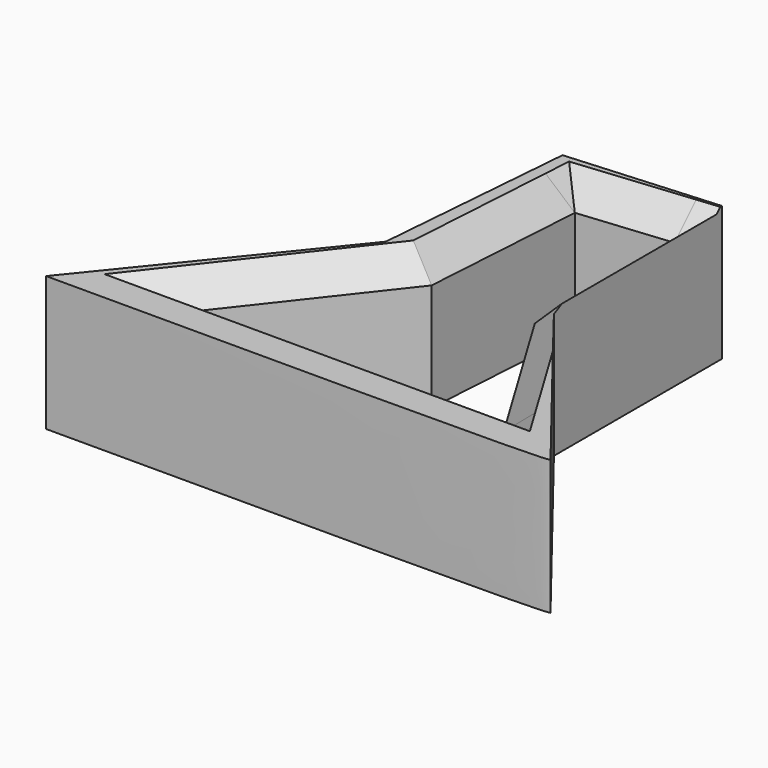
from build123d import *

# Parameters (mm, degrees)
F1_DEPTH     = 25.4
F3_DEPTH     = 50.8
F5_T4_DEPTH  = 64.0057067986
F5_T9_DEPTH  = 86.9283653755
F5_T15_DEPTH = 60.9737188004
F5_T20_DEPTH = 59.1061688919
F5_T25_DEPTH = 43.6640606018
F5_T31_DEPTH = 57.4502846001


# Not quite as in the source:
# - a fillet or chamfer that OpenCascade refuses, or shapes differently, is made with other operations: its cross-section is extruded or revolved along the edge and cut away or added
# - a feature of the source that left no trace in its solid (it failed there, or was rolled back) is left out


with BuildPart() as f1:
    # F0 (on Top) → F1 (new body)
    with BuildSketch(Plane.XY):
        with BuildLine():
            add(Edge.make_bspline(
                [(-48.315115273, -59.7526505589), (-37.5784229901, -46.4742837681), (-26.8417307072, -33.1959169772), (-16.1050384243, -19.9175501863)],
                knots=[0, 0, 0, 0, 51.2281589782, 51.2281589782, 51.2281589782, 51.2281589782], degree=3))
            add(Edge.make_bspline(
                [(-48.315115273, -59.7526505589), (-1.0274761031, -59.7958142001), (46.2601630669, -59.8389778412), (46.3316738605, -59.1182820499)],
                knots=[0, 0, 0, 0, 0.8911107377, 0.8911107377, 0.8911107377, 0.8911107377], degree=3))
            add(Edge.make_bspline(
                [(46.3316738605, -59.1182820499), (46.3235373894, -59.1079000767), (46.3154009182, -59.0975181035), (46.3072644471, -59.0871361303)],
                knots=[0, 0, 0, 0, 0.0395712999, 0.0395712999, 0.0395712999, 0.0395712999], degree=3))
            add(Edge.make_bspline(
                [(46.3072644471, -59.0871361303), (36.0194733937, -45.9601220924), (25.7316823403, -32.8331080545), (15.4438912868, -19.7060940166)],
                knots=[0.0395712999, 0.0395712999, 0.0395712999, 0.0395712999, 50.0737024584, 50.0737024584, 50.0737024584, 50.0737024584], degree=3))
            add(Edge.make_bspline(
                [(15.4438912868, -19.7060940166), (10.2959275246, -13.1373960111), (5.1479637623, -6.5686980055), (0, 0)],
                knots=[50.0737024584, 50.0737024584, 50.0737024584, 50.0737024584, 75.1105536876, 75.1105536876, 75.1105536876, 75.1105536876], degree=3))
            add(Edge.make_bspline(
                [(-16.1050384243, -19.9175501863), (-10.7366922829, -13.2783667909), (-5.3683461414, -6.6391833954), (0, 0)],
                knots=[51.2281589782, 51.2281589782, 51.2281589782, 51.2281589782, 76.8422384673, 76.8422384673, 76.8422384673, 76.8422384673], degree=3))
        make_face()
        with BuildLine():
            add(Edge.make_bspline(
                [(-16.1050384243, -19.9175501863), (-15.0708617229, -7.3149574714), (-14.0366850214, 5.2876352436), (-13.0025083199, 17.8902279586)],
                knots=[0, 0, 0, 0, 37.9348623472, 37.9348623472, 37.9348623472, 37.9348623472], degree=3))
            add(Edge.make_bspline(
                [(-16.1050384243, -19.9175501863), (-10.7366922829, -13.2783667909), (-5.3683461414, -6.6391833954), (0, 0)],
                knots=[51.2281589782, 51.2281589782, 51.2281589782, 51.2281589782, 76.8422384673, 76.8422384673, 76.8422384673, 76.8422384673], degree=3))
            add(Edge.make_bspline(
                [(15.4438912868, -19.7060940166), (10.2959275246, -13.1373960111), (5.1479637623, -6.5686980055), (0, 0)],
                knots=[50.0737024584, 50.0737024584, 50.0737024584, 50.0737024584, 75.1105536876, 75.1105536876, 75.1105536876, 75.1105536876], degree=3))
            add(Edge.make_bspline(
                [(15.4438912868, -19.7060940166), (15.4438912868, -6.5000866436), (15.4438912868, 6.7059207294), (15.4438912868, 19.9119281024)],
                knots=[0, 0, 0, 0, 39.618022119, 39.618022119, 39.618022119, 39.618022119], degree=3))
            add(Edge.make_bspline(
                [(15.4438912868, 19.9119281024), (5.9617580846, 19.2380280544), (-3.5203751177, 18.5641280065), (-13.0025083199, 17.8902279586)],
                knots=[0, 0, 0, 0, 28.5181507475, 28.5181507475, 28.5181507475, 28.5181507475], degree=3))
        make_face()
    extrude(amount=F1_DEPTH)

    # F2 (on Top) → F3 (cut)
    with BuildSketch(Plane.XY):
        with BuildLine():
            add(Edge.make_bspline(
                [(11.2517978996, 14.0004176646), (5.4347412661, 13.426968207), (-0.3823153675, 12.8535187493), (-6.199372001, 12.2800692916)],
                knots=[0, 0, 0, 0, 17.5357614441, 17.5357614441, 17.5357614441, 17.5357614441], degree=3))
            add(Edge.make_bspline(
                [(-6.199372001, 12.2800692916), (-6.8688768273, 1.8608955046), (-7.5383816535, -8.5582782825), (-8.2078864798, -18.9774520695)],
                knots=[0, 0, 0, 0, 31.3219854424, 31.3219854424, 31.3219854424, 31.3219854424], degree=3))
            add(Edge.make_bspline(
                [(-8.2078864798, -18.9774520695), (-15.9868902216, -28.9221989612), (-23.7658939635, -38.8669458528), (-31.5448977053, -48.8116927445)],
                knots=[0, 0, 0, 0, 37.8774076409, 37.8774076409, 37.8774076409, 37.8774076409], degree=3))
            add(Edge.make_bspline(
                [(-31.5448977053, -48.8116927445), (-14.2238239447, -48.8116927445), (3.0972498159, -48.8116927445), (20.4183235765, -48.8116927445)],
                knots=[0, 0, 0, 0, 51.9632212818, 51.9632212818, 51.9632212818, 51.9632212818], degree=3))
            add(Edge.make_bspline(
                [(20.4183235765, -48.8116927445), (23.3639385551, -48.8116927445), (26.3095535338, -48.8116927445), (29.2551685125, -48.8116927445)],
                knots=[0, 0, 0, 0, 8.836844936, 8.836844936, 8.836844936, 8.836844936], degree=3))
            add(Edge.make_bspline(
                [(29.2551685125, -48.8116927445), (23.2540449748, -38.8669458528), (17.2529214372, -28.9221989612), (11.2517978996, -18.9774520695)],
                knots=[0, 0, 0, 0, 34.8454196427, 34.8454196427, 34.8454196427, 34.8454196427], degree=3))
            add(Edge.make_bspline(
                [(11.2517978996, -18.9774520695), (11.2517978996, -7.9848288248), (11.2517978996, 3.0077944199), (11.2517978996, 14.0004176646)],
                knots=[0, 0, 0, 0, 32.9778697342, 32.9778697342, 32.9778697342, 32.9778697342], degree=3))
        make_face()
    extrude(amount=F3_DEPTH, mode=Mode.SUBTRACT)

    # F5: chamfer of 5.08 on 6 edges, made by hand


with BuildPart() as f5_tool2:
    # F5_s3 → F5_t4 (new body)
    with BuildSketch(Plane(origin=(-43.7113633895, -55.8809919142, 0), x_dir=(0, 0, 1), z_dir=(0.6161195467, 0.7876526545, 0))):
        Polygon((25.4, 0.1474155925), (20.32, 5.2274155925), (25.4, 5.2274155925), align=None)
    extrude(amount=F5_T4_DEPTH)

    split(bisect_by=Plane(origin=(0, -14.2458463722, -14.2458463722), x_dir=(1, 0, 0), z_dir=(0, 0.7071067812, 0.7071067812)), keep=Keep.TOP)


with BuildPart() as f1_1:
    add(f1.part)

    # F5_t1: cut F5_tool2
    add(f5_tool2.part, mode=Mode.SUBTRACT)


with BuildPart() as f5_tool7:
    # F5_s8 → F5_t9 (new body)
    with BuildSketch(Plane.YZ.offset(-44.6090472842)):
        Polygon((-53.8916927445, 25.4), (-48.8116927445, 20.32), (-48.8116927445, 25.4), align=None)
    extrude(amount=F5_T9_DEPTH)

    split(bisect_by=Plane(origin=(-8.7722085747, -5.293559296, 10.2456533856), x_dir=(0.5166639058, -0.856188302, 0), z_dir=(-0.6054165543, -0.3653365514, 0.7071067812)), keep=Keep.TOP)

    split(bisect_by=Plane(origin=(10.0612448539, -7.870131057, 12.7737077963), x_dir=(0.6161195467, 0.7876526545, 0), z_dir=(0.5569545332, -0.4356623095, 0.7071067812)), keep=Keep.TOP)


with BuildPart() as f1_2:
    add(f1_1.part)

    # F5_t6: cut F5_tool7
    add(f5_tool7.part, mode=Mode.SUBTRACT)


with BuildPart() as f5_tool13:
    # F5_s14 → F5_t15 (new body)
    with BuildSketch(Plane(origin=(4.6486942055, -7.7035719995, 0), x_dir=(0, 0, 1), z_dir=(0.5166639058, -0.856188302, 0))):
        Polygon((25.4, -4.9086932287), (20.32, 0.1713067713), (25.4, 0.1713067713), align=None)
    extrude(amount=F5_T15_DEPTH)

    split(bisect_by=Plane(origin=(0, -14.2458463722, -14.2458463722), x_dir=(1, 0, 0), z_dir=(0, 0.7071067812, 0.7071067812)), keep=Keep.TOP)


with BuildPart() as f1_3:
    add(f1_2.part)

    # F5_t12: cut F5_tool13
    add(f5_tool13.part, mode=Mode.SUBTRACT)


with BuildPart() as f5_tool18:
    # F5_s19 → F5_t20 (new body)
    with BuildSketch(Plane.XZ.offset(-27.0645672435)):
        Polygon((16.3317978996, 25.4), (11.2517978996, 20.32), (11.2517978996, 25.4), align=None)
    extrude(amount=F5_T20_DEPTH)

    split(bisect_by=Plane(origin=(0.3674517714, -3.7274213716, 3.7454894054), x_dir=(0.9951760553, 0.0981051424, 0), z_dir=(0.0693708114, -0.7036957372, 0.7071067812)), keep=Keep.TOP)


with BuildPart() as f1_4:
    add(f1_3.part)

    # F5_t17: cut F5_tool18
    add(f5_tool18.part, mode=Mode.SUBTRACT)


with BuildPart() as f5_tool23:
    # F5_s24 → F5_t25 (new body)
    with BuildSketch(Plane(origin=(-17.9419078945, -1.7687256632, 0), x_dir=(0, 0, 1), z_dir=(0.9951760553, 0.0981051424, 0))):
        Polygon((25.4, -17.9090211892), (20.32, -12.8290211892), (25.4, -12.8290211892), align=None)
    extrude(amount=F5_T25_DEPTH)

    split(bisect_by=Plane(origin=(6.6592316135, -0.4279022306, 6.672965308), x_dir=(0.0641247498, 0.9979418903, 0), z_dir=(0.7056514779, -0.0453430454, 0.7071067812)), keep=Keep.TOP)

    split(bisect_by=Plane(origin=(-4.5341010502, 0, 4.5341010502), x_dir=(0, 1, 0), z_dir=(-0.7071067812, 0, 0.7071067812)), keep=Keep.TOP)


with BuildPart() as f1_5:
    add(f1_4.part)

    # F5_t22: cut F5_tool23
    add(f5_tool23.part, mode=Mode.SUBTRACT)


with BuildPart() as f5_tool29:
    # F5_s30 → F5_t31 (new body)
    with BuildSketch(Plane(origin=(-2.0859058182, -32.4619246499, 0), x_dir=(0, 0, 1), z_dir=(0.0641247498, 0.9979418903, 0))):
        Polygon((25.4, -12.054069384), (20.32, -6.974069384), (25.4, -6.974069384), align=None)
    extrude(amount=F5_T31_DEPTH)

    split(bisect_by=Plane(origin=(0.3674517714, -3.7274213716, 3.7454894054), x_dir=(0.9951760553, 0.0981051424, 0), z_dir=(0.0693708114, -0.7036957372, 0.7071067812)), keep=Keep.TOP)


with BuildPart() as f1_6:
    add(f1_5.part)

    # F5_t28: cut F5_tool29
    add(f5_tool29.part, mode=Mode.SUBTRACT)


solid = f1_6.part
